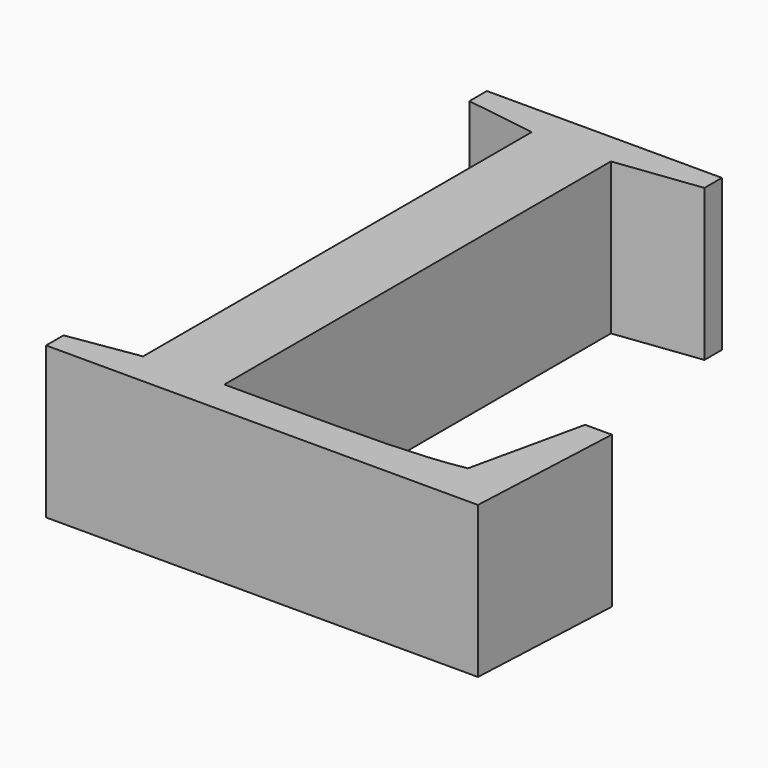
from build123d import *

# Parameters (mm, degrees)
F0_TEXT_SIZE = 17.6388888889
F1_DEPTH     = 3.175


# Not quite as in the source:
# - Text() gives the source's letters only with a copy of the font that has no kerning and outlines rounded to 1/6400 em; it was checked with that copy


with BuildPart() as f1:
    # F0 (on Top) → F1 (new body)
    with BuildSketch(Plane.XY):
        with Locations((-72.8042222081, 58.62646054)):
            Text('L', F0_TEXT_SIZE, font='Tinos', text_align=(TextAlign.LEFT, TextAlign.BOTTOM))
    extrude(amount=F1_DEPTH)


solid = f1.part
